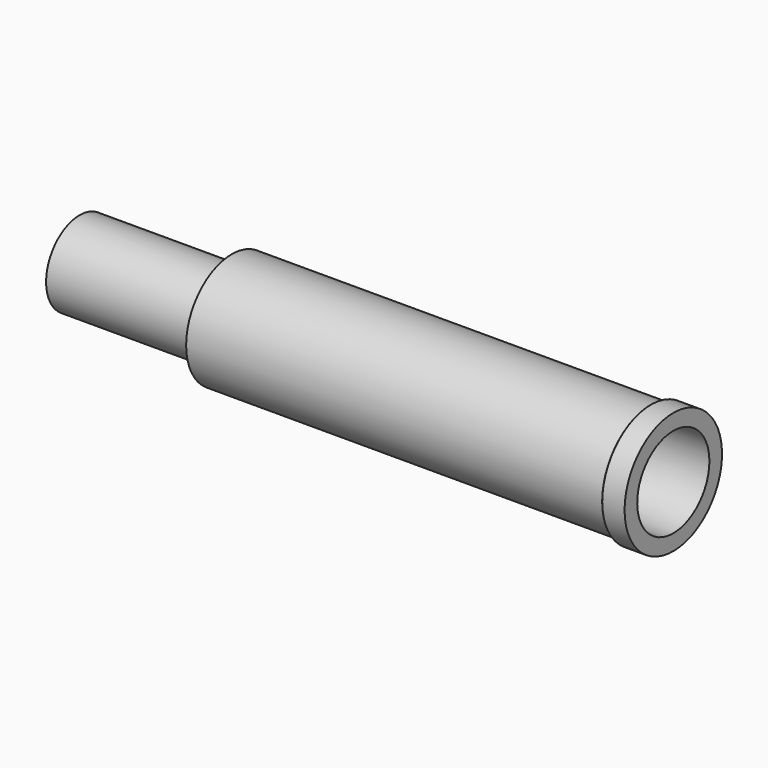
from build123d import *

# Parameters (mm, degrees)
F2_W = 100
F2_H = 6.1
F5_R = 0.2


# Not quite as in the source:
# - a feature of the source that left no trace in its solid (it failed there, or was rolled back) is left out


with BuildPart() as f1:
    # F0 (on Top) → F1 (revolve)
    with BuildSketch(Plane.XY):
        Polygon((53, -16), (53, 0), (47, 0), (0, 0), (-103, 0), (-103, -11), (-63, -11), (-63, -15), (47, -15), (47, -16), align=None)
    revolve(axis=Axis((-51.5, 0, 0), (-1, 0, 0)))

    # F2 (on Front) → F3 (revolve, cut)
    with BuildSketch(Plane.XZ):
        Polygon((53, 11.85), (-34, 9.6771213406), (-34, 6.1), (-34, 0), (0, 0), (53, 0), align=None)
        with Locations((-84, 3.05)):
            Rectangle(F2_W, F2_H)
    revolve(axis=Axis((26.5, 0, 0), (-1, 0, 0)), mode=Mode.SUBTRACT)

    # F5
    f5_edges = [f1.edges().sort_by_distance(p)[0] for p in [
        (47, 16, 0),
        (47, 15, 0),
    ]]
    fillet(f5_edges, radius=F5_R)


solid = f1.part
